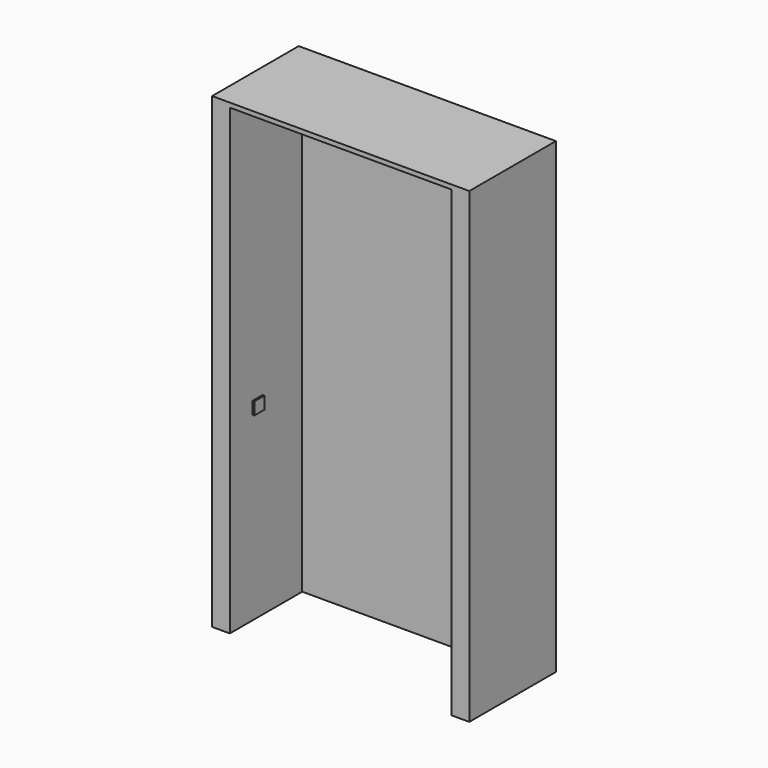
from build123d import *

# Parameters (mm, degrees)
F1_DEPTH = 2610
F2_W     = 1450
F2_H     = 610
F3_DEPTH = 25
F5_W     = 70
F5_H     = 70
F6_DEPTH = 104
F7_DEPTH = 10
F8_W     = 70
F8_H     = 70
F9_DEPTH = 10


# Not quite as in the source:
# - the program builds the solid bodies; features that only make, move or delete a surface that nothing else refers to are left out


with BuildPart() as f1:
    # F0 (on Top) → F1 (new body)
    with BuildSketch(Plane.XY):
        Polygon((-100, -510), (0, -510), (0, 0), (1250, 0), (1250, -510), (1350, -510), (1350, 100), (-100, 100), align=None)
    extrude(amount=F1_DEPTH)

    # F2 (on face) → F3 (join)
    with BuildSketch(Plane.XY.offset(2610)):
        with Locations((625, -205)):
            Rectangle(F2_W, F2_H)
    extrude(amount=F3_DEPTH)

    # F5 (on face) → F6 (join)
    with BuildSketch(Plane(origin=(1250, 0, 0), x_dir=(0, -1, 0), z_dir=(-1, 0, 0))):
        with Locations((285, 1075)):
            Rectangle(F5_W, F5_H)
    extrude(amount=F6_DEPTH)

    # F5 (on face) → F7 (join)
    with BuildSketch(Plane(origin=(1250, 0, 0), x_dir=(0, -1, 0), z_dir=(-1, 0, 0))):
        with Locations((203.0151075125, 1915.4621696472)):
            Rectangle(F5_W, F5_H)
    extrude(amount=F7_DEPTH)

    # F8 (on face) → F9 (join)
    with BuildSketch(Plane.YZ):
        with Locations((-314.7198361158, 1055)):
            Rectangle(F8_W, F8_H)
    extrude(amount=F9_DEPTH)


solid = f1.part
